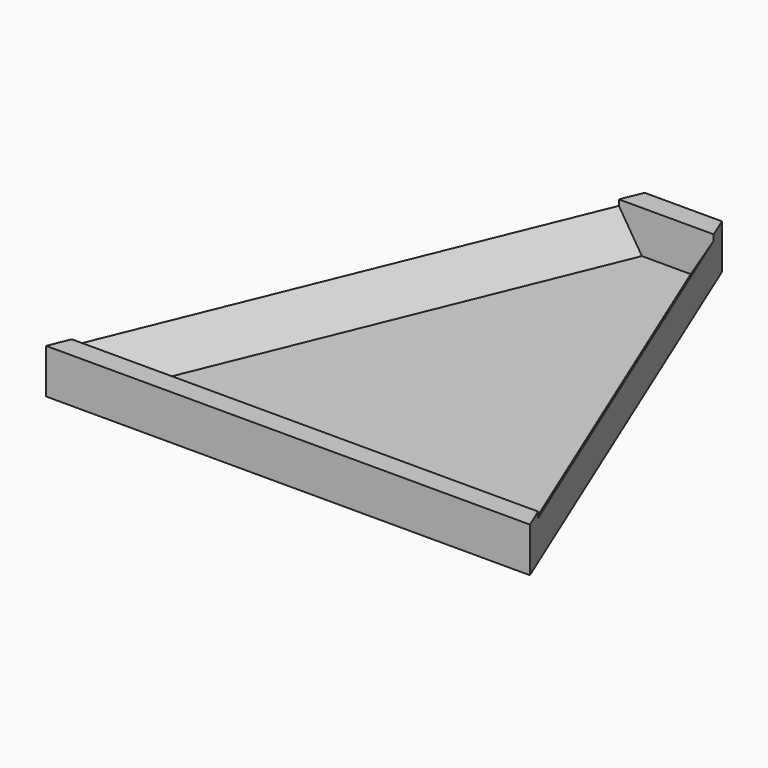
from build123d import *

# Parameters (mm, degrees)
F1_DEPTH     = 9.9999997765
F3_DEPTH     = 200
F4_T4_DEPTH  = 3334.8343018584
F4_T10_DEPTH = 3334.8343018584


# Not quite as in the source:
# - a fillet or chamfer that OpenCascade refuses, or shapes differently, is made with other operations: its cross-section is extruded or revolved along the edge and cut away or added


with BuildPart() as f1:
    # F0 (on Top) → F1 (new body)
    with BuildSketch(Plane.XY):
        Polygon((808.0060526885, 2227.0578271406), (-149.2672159397, -100), (2129.2672159397, -100), (1171.9939473115, 2227.0578271406), align=None)
        Polygon((1980, 0), (0, 0), (875, 2127.0578271406), (1105, 2127.0578271406), align=None, mode=Mode.SUBTRACT)
        Polygon((875, 2127.0578271406), (0, 0), (1980, 0), (1105, 2127.0578271406), align=None)
    extrude(amount=-F1_DEPTH)

    # F2 (on face) → F3 (join)
    with BuildSketch(Plane.XY):
        Polygon((1171.9939473115, 2227.0578271406), (808.0060526885, 2227.0578271406), (-149.2672159397, -100), (2129.2672159397, -100), align=None)
        Polygon((1980, 0), (0, 0), (875, 2127.0578271406), (1105, 2127.0578271406), align=None, mode=Mode.SUBTRACT)
    extrude(amount=F3_DEPTH)

    # F4: chamfer of 200 x 115.4700538379 on 2 edges, made by hand


with BuildPart() as f4_tool2:
    # F4_s3 → F4_t4 (new body)
    with BuildSketch(Plane(origin=(-196.8434813318, -478.5113916438, 0), x_dir=(0, 0, 1), z_dir=(0.3804347826, 0.9248077509, 0))):
        Polygon((200, -115.4700538379), (0, 0), (200, 0), align=None)
    extrude(amount=F4_T4_DEPTH)

    split(bisect_by=Plane.XZ.offset(-2127.0578271406), keep=Keep.TOP)

    split(bisect_by=Plane.XZ, keep=Keep.BOTTOM)


with BuildPart() as f1_1:
    add(f1.part)

    # F4_t1: cut F4_tool2
    add(f4_tool2.part, mode=Mode.SUBTRACT)


with BuildPart() as f4_tool8:
    # F4_s9 → F4_t10 (new body)
    with BuildSketch(Plane(origin=(-785.2768461711, 1908.9477281377, 0), x_dir=(0, 0, 1), z_dir=(0.3804347826, -0.9248077509, 0))):
        Polygon((200, -1946.5894006807), (0, -1831.1193468428), (200, -1831.1193468428), align=None)
    extrude(amount=F4_T10_DEPTH)

    split(bisect_by=Plane.XZ.offset(-2127.0578271406), keep=Keep.TOP)

    split(bisect_by=Plane.XZ, keep=Keep.BOTTOM)


with BuildPart() as f1_2:
    add(f1_1.part)

    # F4_t7: cut F4_tool8
    add(f4_tool8.part, mode=Mode.SUBTRACT)


solid = f1_2.part
